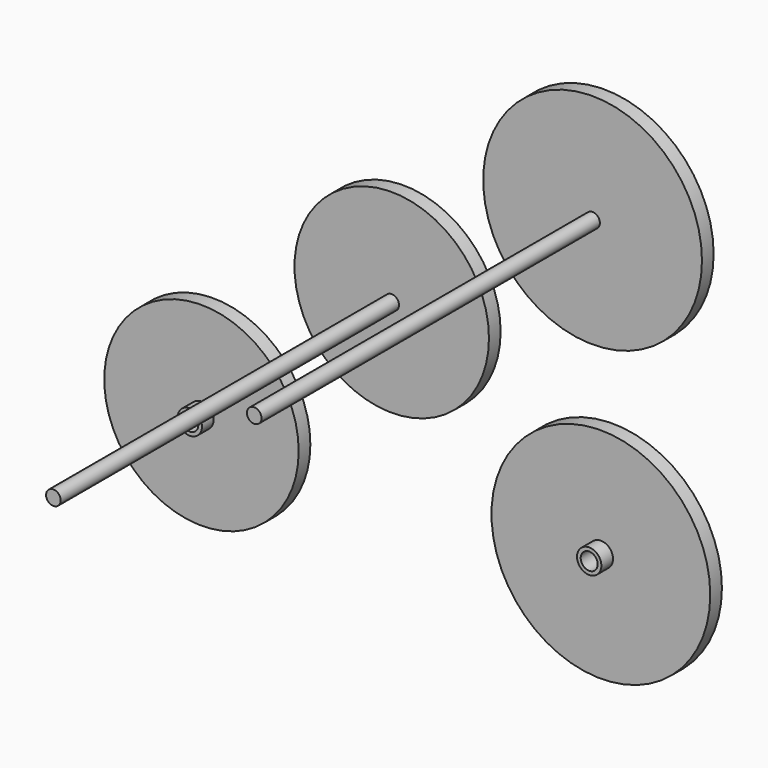
from build123d import *

# Parameters (mm, degrees)
F0_R     = 20
F0_R_2   = 1.5
F1_DEPTH = 3
F0_R_3   = 2.5
F0_R_4   = 22.5
F2_DEPTH = 90
F0_R_5   = 1.75
F3_DEPTH = 6
F4_DEPTH = 90


# Not quite as in the source:
# - a feature names something its author has since deleted; it is built from what else it names


with BuildPart() as f1:
    # F0 (on Front) → F1 (new body)
    with BuildSketch(Plane.XZ):
        Circle(F0_R)
        Circle(F0_R_2, mode=Mode.SUBTRACT)
    extrude(amount=F1_DEPTH)

    # F0 (on Front) → F2 (join)
    with BuildSketch(Plane.XZ):
        Circle(F0_R_2)
    extrude(amount=F2_DEPTH)


with BuildPart() as f1b:
    # F0 (on Front) → F1, piece 2 (new body)
    with BuildSketch(Plane.XZ):
        with Locations((-39.1355007887, -33.1673398614)):
            Circle(F0_R)
        with Locations((-39.1355007887, -33.1673398614)):
            Circle(F0_R_3, mode=Mode.SUBTRACT)
    extrude(amount=F1_DEPTH)

    # F0 (on Front) → F3 (join)
    with BuildSketch(Plane.XZ):
        with Locations((-39.1355007887, -33.1673398614)):
            Circle(F0_R_3)
        with Locations((-39.1355007887, -33.1673398614)):
            Circle(F0_R_5, mode=Mode.SUBTRACT)
    extrude(amount=F3_DEPTH)


with BuildPart() as f1c:
    # F0 (on Front) → F1, piece 3 (new body)
    with BuildSketch(Plane.XZ):
        with Locations((43.018873781, -31.6528305411)):
            Circle(F0_R_4)
        with Locations((43.018873781, -31.6528305411)):
            Circle(F0_R_3, mode=Mode.SUBTRACT)
    extrude(amount=F1_DEPTH)

    # F0 (on Front) → F3, piece 2 (join)
    with BuildSketch(Plane.XZ):
        with Locations((43.018873781, -31.6528305411)):
            Circle(F0_R_3)
        with Locations((43.018873781, -31.6528305411)):
            Circle(F0_R_5, mode=Mode.SUBTRACT)
    extrude(amount=F3_DEPTH)


with BuildPart() as f1d:
    # F0 (on Front) → F1, piece 4 (new body)
    with BuildSketch(Plane.XZ):
        with Locations((41.3147807121, 28.3098872751)):
            Circle(F0_R_4)
        with Locations((41.3147807121, 28.3098872751)):
            Circle(F0_R_2, mode=Mode.SUBTRACT)
    extrude(amount=F1_DEPTH)

    # F0 (on Front) → F4 (join)
    with BuildSketch(Plane.XZ):
        with Locations((41.3147807121, 28.3098872751)):
            Circle(F0_R_2)
    extrude(amount=F4_DEPTH)


solid = Compound([f1.part, f1b.part, f1c.part, f1d.part])
